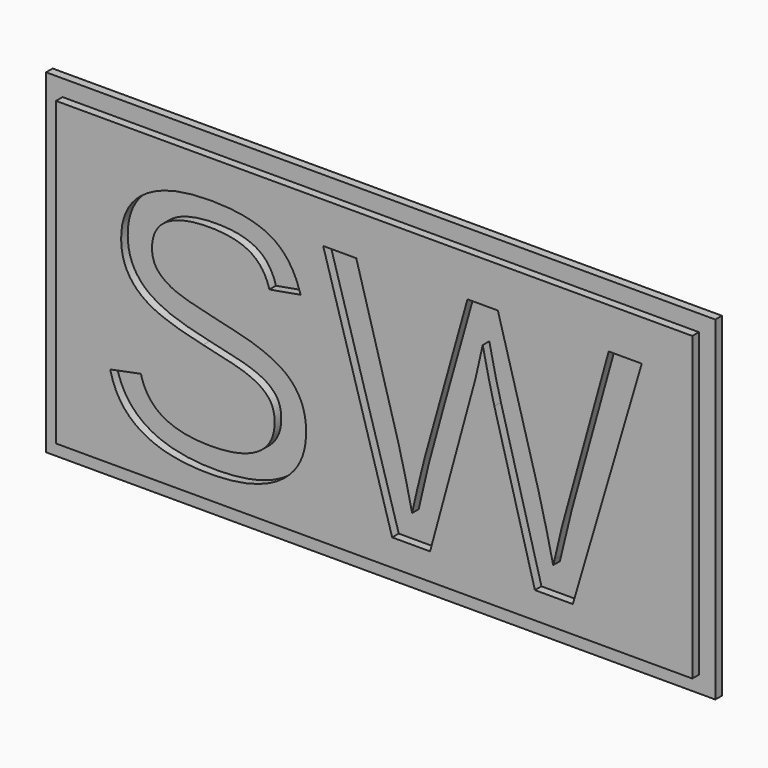
from build123d import *

# Parameters (mm, degrees)
F0_W         = 203.25
F0_H         = 101.6
F0_W_2       = 193.25
F0_H_2       = 91.6
F1_DEPTH     = 2.5
F2_DEPTH     = 2.5
F3_TEXT_SIZE = 103.3482646259
F4_DEPTH     = 2.6


# Not quite as in the source:
# - Text() gives the source's letters only with a copy of the font that has no kerning and outlines rounded to 1/6400 em; it was checked with that copy


with BuildPart() as f1:
    # F0 (on Front) → F1 (new body)
    with BuildSketch(Plane.XZ):
        with Locations((101.625, 50.8)):
            Rectangle(F0_W, F0_H)
        with Locations((101.625, 50.8)):
            Rectangle(F0_W_2, F0_H_2, mode=Mode.SUBTRACT)
        with Locations((101.625, 50.8)):
            Rectangle(F0_W_2, F0_H_2)
    extrude(amount=-F1_DEPTH)


with BuildPart() as f2:
    # F0 (on Front) → F2 (new body)
    with BuildSketch(Plane.XZ):
        with Locations((101.625, 50.8)):
            Rectangle(F0_W_2, F0_H_2)
    extrude(amount=F2_DEPTH)

    # F3 (on face) → F4 (cut)
    with BuildSketch(Plane.XZ.offset(2.5)):
        with Locations((16.772704199, 13.0987772718)):
            Text('SW', F3_TEXT_SIZE, font='Arimo', text_align=(TextAlign.LEFT, TextAlign.BOTTOM))
    extrude(amount=-F4_DEPTH, mode=Mode.SUBTRACT)


solid = Compound([f1.part, f2.part])
